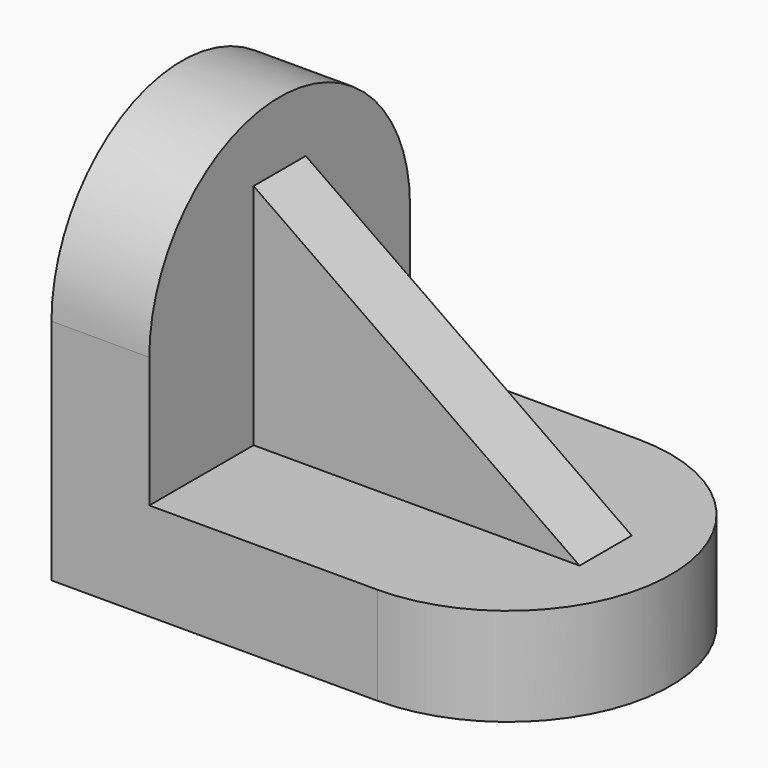
from build123d import *

# Parameters (mm, degrees)
F1_DEPTH = 1270
F3_DEPTH = 381
F5_DEPTH = 381
F7_START = -508
F7_DEPTH = 254


# Not quite as in the source:
# - a feature names something its author has since deleted; it is built from what else it names


with BuildPart() as f1:
    # F0 (on Front) → F1 (new body)
    with BuildSketch(Plane.XZ):
        Polygon((0, 889), (0, 0), (1270, 0), (1270, 381), (381, 381), (381, 889), align=None)
    extrude(amount=F1_DEPTH)

    # F2 (on face) → F3 (join, through all)
    with BuildSketch(Plane.YZ.offset(381)):
        with BuildLine():
            Line((-1270, 889), (0, 889))
            ThreePointArc((0, 889), (-635, 1524), (-1270, 889))
        make_face()
    extrude(amount=-F3_DEPTH)

    # F4 (on face) → F5 (join, through all)
    with BuildSketch(Plane.XY.offset(381)):
        with BuildLine():
            Line((1270, 0), (1270, -1270))
            ThreePointArc((1270, -1270), (1905, -635), (1270, 0))
        make_face()
    extrude(amount=-F5_DEPTH)


with BuildPart() as f7:
    # F6 (on face) → F7 (new body)
    with BuildSketch(Plane.XZ.offset(1270).offset(F7_START)):
        Polygon((1651, 381), (381, 1270), (381, 889), (381, 381), (1270, 381), align=None)
    extrude(amount=-F7_DEPTH)


solid = Compound([f1.part, f7.part])
